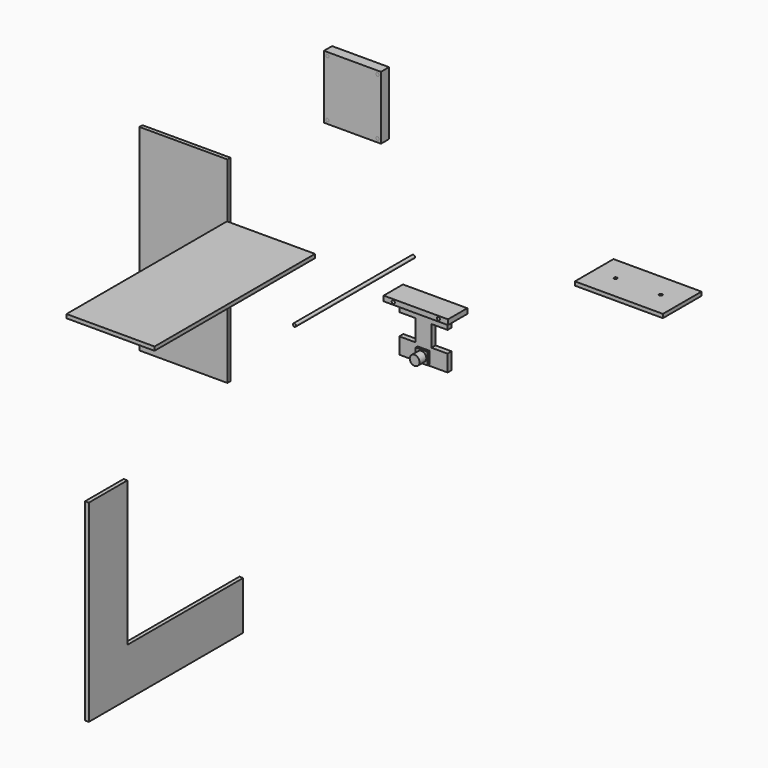
from build123d import *

# Parameters (mm, degrees)
F0_W      = 101.6
F0_H      = 8
F0_R      = 2.5
F1_DEPTH  = 38.1
F2_R      = 2.5
F3_DEPTH  = 234.6
F5_DEPTH  = 6
F6_W      = 138.99896
F6_H      = 310.7944
F7_DEPTH  = 6
F8_W      = 139
F8_H      = 316.8
F9_DEPTH  = 6
F10_W     = 139
F10_H     = 76.2
F10_R     = 2.5
F11_DEPTH = 6
F12_W     = 90
F12_H     = 100
F12_R     = 2.5
F13_DEPTH = 16
F14_DEPTH = 16
F15_W     = 76.2
F15_H     = 8
F16_DEPTH = 76.2
F17_W     = 25.4
F17_H     = 32.9780355096
F17_H_2   = 33.673774451
F18_DEPTH = 676.0766565222
F17_W_2   = 18.7849588692
F17_H_3   = 18.7849588692
F17_R     = 7.7239634119
F19_DEPTH = 12
F17_R_2   = 5.4539048991
F20_DEPTH = 25.4


# Not quite as in the source:
# - a feature of the source that left no trace in its solid (it failed there, or was rolled back) is left out


with BuildPart() as f1:
    # F0 (on Front) → F1 (new body)
    with BuildSketch(Plane.XZ):
        Rectangle(F0_W, F0_H)
        with Locations((-35.6, 0)):
            Circle(F0_R, mode=Mode.SUBTRACT)
        with Locations((35.6, 0)):
            Circle(F0_R, mode=Mode.SUBTRACT)
    extrude(amount=F1_DEPTH)

    # F15 (on face) → F16 (join)
    with BuildSketch(Plane(origin=(0, 0, -4), x_dir=(1, 0, 0), z_dir=(0, 0, -1))):
        with Locations((0, 19.05)):
            Rectangle(F15_W, F15_H)
    extrude(amount=F16_DEPTH)

    # F17 (on face) → F18 (cut, through all)
    with BuildSketch(Plane(origin=(0, -15.05, 0), x_dir=(-1, 0, 0), z_dir=(0, 1, 0))):
        with Locations((-25.4, -37.508122623)):
            Rectangle(F17_W, F17_H)
        with Locations((25.4, -37.8559920937)):
            Rectangle(F17_W, F17_H_2)
    extrude(amount=-F18_DEPTH, mode=Mode.SUBTRACT)


with BuildPart() as f3:
    # F2 (on Front) → F3 (new body)
    with BuildSketch(Plane.XZ):
        with Locations((-34.4059243798, 48.2007525861)):
            Circle(F2_R)
    extrude(amount=F3_DEPTH)


with BuildPart() as f5:
    # F4 (on Right) → F5 (new body)
    with BuildSketch(Plane.YZ):
        Polygon((-614.9256565222, -228.6), (-614.9256565222, 0), (-691.1256565222, 0), (-691.1256565222, -304.8), (-386.3256565222, -304.8), (-386.3256565222, -228.6), align=None)
    extrude(amount=F5_DEPTH)


with BuildPart() as f7:
    # F6 (on Front) → F7 (new body)
    with BuildSketch(Plane.XZ):
        with Locations((-392.6940560341, -63.7792117634)):
            Rectangle(F6_W, F6_H)
    extrude(amount=F7_DEPTH)


with BuildPart() as f9:
    # F8 (on Top) → F9 (new body)
    with BuildSketch(Plane.XY):
        with Locations((-253.5598740487, -165.4277235146)):
            Rectangle(F8_W, F8_H)
    extrude(amount=F9_DEPTH)


with BuildPart() as f11:
    # F10 (on Top) → F11 (new body)
    with BuildSketch(Plane.XY):
        with Locations((181.5372826105, 173.9297149658)):
            Rectangle(F10_W, F10_H)
        with Locations((145.9372826105, 173.9297149658)):
            Circle(F10_R, mode=Mode.SUBTRACT)
        with Locations((217.1372826105, 173.9297149658)):
            Circle(F10_R, mode=Mode.SUBTRACT)
    extrude(amount=F11_DEPTH)


with BuildPart() as f13:
    # F12 (on Front) → F13 (new body)
    with BuildSketch(Plane.XZ):
        with Locations((-130.562209487, 238.2797680418)):
            Rectangle(F12_W, F12_H)
        with Locations((-170.062209487, 193.7797680418)):
            Circle(F12_R, mode=Mode.SUBTRACT)
        with Locations((-91.062209487, 193.7797680418)):
            Circle(F12_R, mode=Mode.SUBTRACT)
        with Locations((-170.062209487, 282.7797680418)):
            Circle(F12_R, mode=Mode.SUBTRACT)
        with Locations((-91.062209487, 282.7797680418)):
            Circle(F12_R, mode=Mode.SUBTRACT)
    extrude(amount=-F13_DEPTH)


with BuildPart() as f14:
    # F12 (on Front) → F14 (new body)
    with BuildSketch(Plane.XZ):
        with Locations((-170.062209487, 282.7797680418)):
            Circle(F12_R)
    extrude(amount=-F14_DEPTH)


with BuildPart() as f14b:
    # F12 (on Front) → F14, piece 2 (new body)
    with BuildSketch(Plane.XZ):
        with Locations((-91.062209487, 282.7797680418)):
            Circle(F12_R)
    extrude(amount=-F14_DEPTH)


with BuildPart() as f14c:
    # F12 (on Front) → F14, piece 3 (new body)
    with BuildSketch(Plane.XZ):
        with Locations((-91.062209487, 193.7797680418)):
            Circle(F12_R)
    extrude(amount=-F14_DEPTH)


with BuildPart() as f14d:
    # F12 (on Front) → F14, piece 4 (new body)
    with BuildSketch(Plane.XZ):
        with Locations((-170.062209487, 193.7797680418)):
            Circle(F12_R)
    extrude(amount=-F14_DEPTH)


with BuildPart() as f19:
    # F17 (on face) → F19 (new body)
    with BuildSketch(Plane(origin=(0, -15.05, 0), x_dir=(-1, 0, 0), z_dir=(0, 1, 0))):
        with Locations((0, -68.6076581478)):
            Rectangle(F17_W_2, F17_H_3)
        with Locations((0, -68.6076581478)):
            Circle(F17_R, mode=Mode.SUBTRACT)
    extrude(amount=-F19_DEPTH)


with BuildPart() as f20:
    # F17 (on face) → F20 (new body)
    with BuildSketch(Plane(origin=(0, -15.05, 0), x_dir=(-1, 0, 0), z_dir=(0, 1, 0))):
        with Locations((0, -68.6076581478)):
            Circle(F17_R)
        with Locations((0, -68.6076581478)):
            Circle(F17_R_2, mode=Mode.SUBTRACT)
        with Locations((0, -68.6076581478)):
            Circle(F17_R_2)
    extrude(amount=-F20_DEPTH)


solid = Compound([f1.part, f3.part, f5.part, f7.part, f9.part, f11.part, f13.part, f14.part, f14b.part, f14c.part, f14d.part, f19.part, f20.part])
